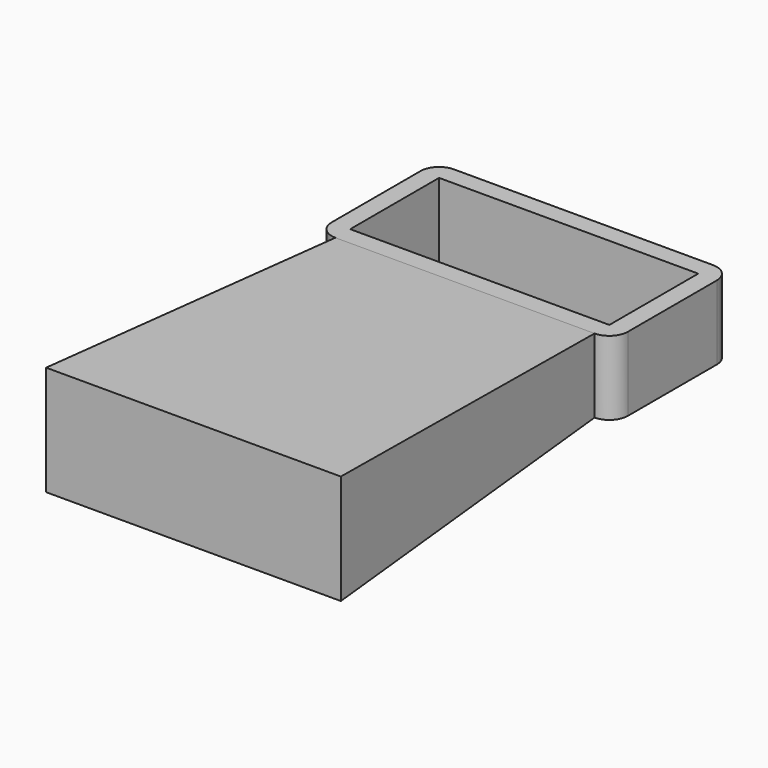
from build123d import *

# Parameters (mm, degrees)
F0_W     = 177.8
F0_H     = 76.2
F1_DEPTH = 50.8
F2_W     = 177.8
F2_H     = 50.8
F3_DEPTH = 232.8048453
F3_TAPER = -3


# Not quite as in the source:
# - an extrude ends at something that could not be found from the text; its depth is read off the source's solid


with BuildPart() as f1:
    # F0 (on Top) → F1 (new body)
    with BuildSketch(Plane.XY):
        with BuildLine():
            ThreePointArc((101.6, 38.1), (97.8802561211, 47.0802561211), (88.9, 50.8))
            Line((88.9, 50.8), (-88.9, 50.8))
            ThreePointArc((-88.9, 50.8), (-97.8802561211, 47.0802561211), (-101.6, 38.1))
            Line((-101.6, 38.1), (-101.6, -38.1))
            ThreePointArc((-101.6, -38.1), (-97.8802561211, -47.0802561211), (-88.9, -50.8))
            Line((-88.9, -50.8), (88.9, -50.8))
            ThreePointArc((88.9, -50.8), (97.8802561211, -47.0802561211), (101.6, -38.1))
            Line((101.6, -38.1), (101.6, 38.1))
        make_face()
        Rectangle(F0_W, F0_H, mode=Mode.SUBTRACT)
    extrude(amount=F1_DEPTH)

    # F2 (on face) → F3 (join, through all)
    with BuildSketch(Plane.XZ.offset(50.8)):
        with Locations((0, 25.4)):
            Rectangle(F2_W, F2_H)
    extrude(amount=F3_DEPTH, taper=F3_TAPER)


solid = f1.part
